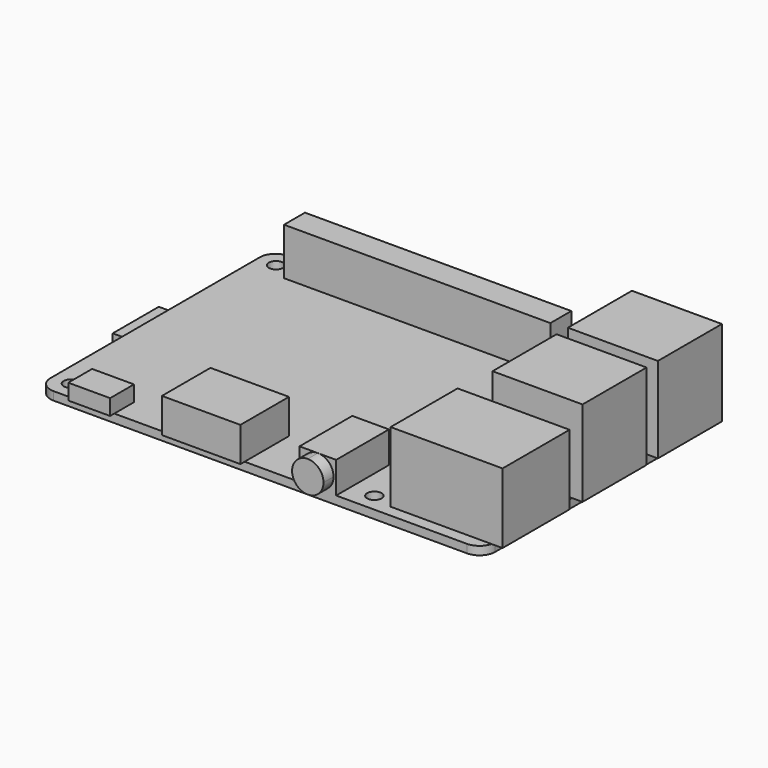
from build123d import *

# Parameters (mm, degrees)
F0_W         = 85
F0_H         = 56
F1_DEPTH     = 1.6
F2_W         = 21.4
F2_H         = 16
F3_DEPTH     = 13.4
F4_W         = 17.2
F4_H         = 15.3
F5_DEPTH     = 16.4
F6_W         = 15
F6_H         = 11.6
F7_DEPTH     = 6.6
F8_W         = 7
F8_H         = 15
F9_DEPTH     = 6
F10_W        = 8
F10_H        = 5.7
F11_DEPTH    = 3
F12_W        = 17
F12_H        = 11
F13_DEPTH    = 1.5
F14_R        = 1.375
F15_DEPTH    = 3.101
F16_T1_DEPTH = 16.6
F16_T3_DEPTH = 9.1
F17_W        = 50.9
F17_H        = 5
F18_DEPTH    = 9
F20_DEPTH    = 2.4


# Not quite as in the source:
# - a fillet or chamfer that OpenCascade refuses, or shapes differently, is made with other operations: its cross-section is extruded or revolved along the edge and cut away or added


with BuildPart() as f1:
    # F0 (on Top) → F1 (new body)
    with BuildSketch(Plane.XY):
        Rectangle(F0_W, F0_H)
    extrude(amount=F1_DEPTH)

    # F2 (on face) → F3 (join)
    with BuildSketch(Plane.XY.offset(1.6)):
        with Locations((33.8, -17.75)):
            Rectangle(F2_W, F2_H)
    extrude(amount=F3_DEPTH)

    # F4 (on face) → F5 (join)
    with BuildSketch(Plane.XY.offset(1.6)):
        with Locations((35.9, 1)):
            Rectangle(F4_W, F4_H)
        with Locations((35.9, 19)):
            Rectangle(F4_W, F4_H)
    extrude(amount=F5_DEPTH)

    # F6 (on face) → F7 (join)
    with BuildSketch(Plane.XY.offset(1.6)):
        with Locations((-10.5, -23.2)):
            Rectangle(F6_W, F6_H)
    extrude(amount=F7_DEPTH)

    # F8 (on face) → F9 (join)
    with BuildSketch(Plane.XY.offset(1.6)):
        with Locations((11, -22.9)):
            Rectangle(F8_W, F8_H)
    extrude(amount=F9_DEPTH)

    # F10 (on face) → F11 (join)
    with BuildSketch(Plane.XY.offset(1.6)):
        with Locations((-31.9, -26.15)):
            Rectangle(F10_W, F10_H)
    extrude(amount=F11_DEPTH)

    # F12 (on face) → F13 (join)
    with BuildSketch(Plane(origin=(0, 0, 0), x_dir=(1, 0, 0), z_dir=(0, 0, -1))):
        with Locations((-37.7, 0)):
            Rectangle(F12_W, F12_H)
    extrude(amount=F13_DEPTH)

    # F14 (on face) → F15 (cut, through all)
    with BuildSketch(Plane.XY.offset(1.6)):
        with Locations((-39, -24.5)):
            Circle(F14_R)
        with Locations((19, -24.5)):
            Circle(F14_R)
        with Locations((-39, 24.5)):
            Circle(F14_R)
        with Locations((19, 24.5)):
            Circle(F14_R)
    extrude(amount=-F15_DEPTH, mode=Mode.SUBTRACT)

    # F16: fillet of radius 3 on 4 edges, made by hand

    # F16_s2 → F16_t1 (cut)
    with BuildSketch(Plane.XY.offset(-7.5)):
        with BuildLine():
            ThreePointArc((-39.5, -28), (-41.6213203436, -27.1213203436), (-42.5, -25))
            Line((-42.5, -25), (-42.5, -28))
            Line((-42.5, -28), (-39.5, -28))
        make_face()
        with BuildLine():
            ThreePointArc((-42.5, 25), (-41.6213203436, 27.1213203436), (-39.5, 28))
            Line((-39.5, 28), (-42.5, 28))
            Line((-42.5, 28), (-42.5, 25))
        make_face()
    extrude(amount=F16_T1_DEPTH, mode=Mode.SUBTRACT)

    # F16_s4 → F16_t3 (cut)
    with BuildSketch(Plane.XY.offset(-7.5)):
        with BuildLine():
            ThreePointArc((39.5, -28), (41.6213203436, -27.1213203436), (42.5, -25))
            Line((42.5, -25), (42.5, -28))
            Line((42.5, -28), (39.5, -28))
        make_face()
        with BuildLine():
            ThreePointArc((42.5, 25), (41.6213203436, 27.1213203436), (39.5, 28))
            Line((39.5, 28), (42.5, 28))
            Line((42.5, 28), (42.5, 25))
        make_face()
    extrude(amount=F16_T3_DEPTH, mode=Mode.SUBTRACT)

    # F17 (on face) → F18 (join)
    with BuildSketch(Plane.XY.offset(1.6)):
        with Locations((-10, 24.4839084893)):
            Rectangle(F17_W, F17_H)
    extrude(amount=F18_DEPTH)

    # F19 (on face) → F20 (cut)
    with BuildSketch(Plane.XZ.offset(30.4)):
        with BuildLine():
            ThreePointArc((11, 7.6), (13.1213203436, 6.7213203436), (14, 4.6))
            ThreePointArc((14, 4.6), (13.1213203436, 2.4786796564), (11, 1.6))
            Line((11, 1.6), (14.5, 1.6))
            Line((14.5, 1.6), (14.5, 7.6))
            Line((14.5, 7.6), (11, 7.6))
        make_face()
        with BuildLine():
            ThreePointArc((11, 1.6), (8, 4.6), (11, 7.6))
            Line((11, 7.6), (7.5, 7.6))
            Line((7.5, 7.6), (7.5, 1.6))
            Line((7.5, 1.6), (11, 1.6))
        make_face()
    extrude(amount=-F20_DEPTH, mode=Mode.SUBTRACT)


solid = f1.part
